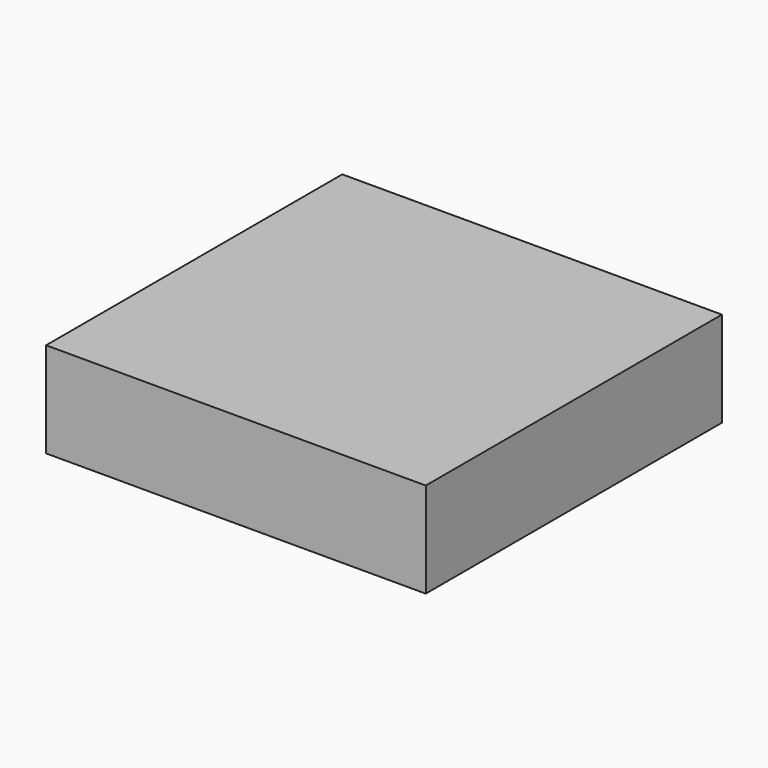
from build123d import *

# Parameters (mm, degrees)
F3_W     = 51.2802042067
F3_H     = 12.8578543663
F4_DEPTH = 25
F5_W     = 51.2802042067
F5_H     = 12.8578543663
F6_DEPTH = 25


# Not quite as in the source:
# - a feature names something its author has since deleted; it is built from what else it names
# - the program builds the solid bodies; features that only make, move or delete a surface that nothing else refers to are left out


with BuildPart() as f4:
    # F3 (on Front) → F4 (new body)
    with BuildSketch(Plane.XZ):
        with Locations((0.2750232816, -6.4289271832)):
            Rectangle(F3_W, F3_H)
    extrude(amount=F4_DEPTH)

    # F5 (on face) → F6 (join)
    with BuildSketch(Plane(origin=(0, 0, 0), x_dir=(-1, 0, 0), z_dir=(0, 1, 0))):
        with Locations((-0.2750232816, -6.4289271832)):
            Rectangle(F5_W, F5_H)
    extrude(amount=F6_DEPTH)


solid = f4.part
